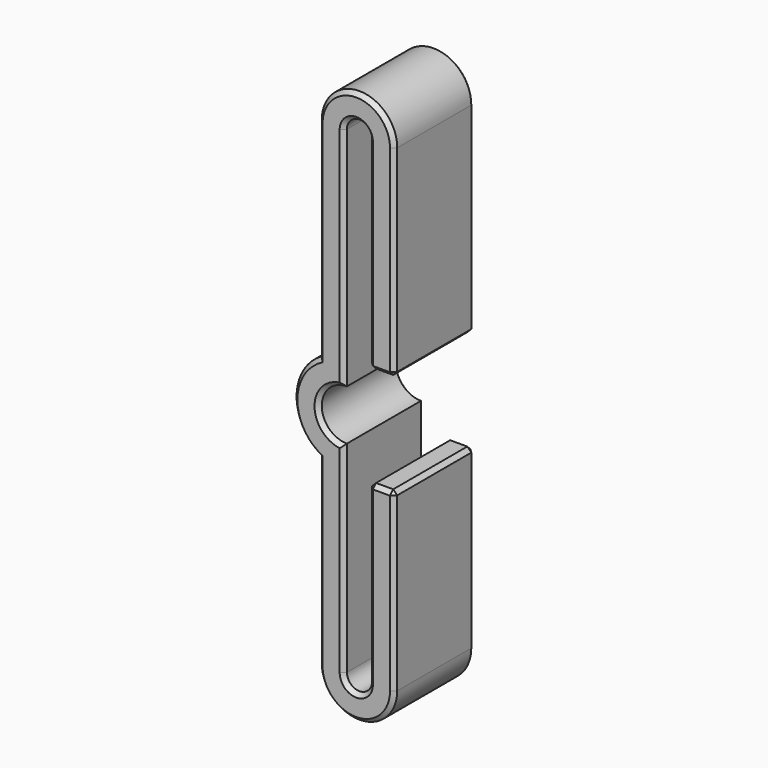
from build123d import *

# Parameters (mm, degrees)
F1_DEPTH = 6.35
F2_SIZE  = 0.254


# Not quite as in the source:
# - a feature names something its author has since deleted; it is built from what else it names


with BuildPart() as f1:
    # F0 (on Front) → F1 (new body)
    with BuildSketch(Plane.XZ):
        with BuildLine():
            Line((0, 1.5875), (0, 15.875))
            ThreePointArc((0, 15.875), (0.79375, 16.66875), (1.5875, 15.875))
            Line((1.5875, 15.875), (1.5875, 3.175))
            Line((1.5875, 3.175), (3.175, 3.175))
            Line((3.175, 3.175), (3.175, 15.875))
            ThreePointArc((3.175, 15.875), (0.79375, 18.25625), (-1.5875, 15.875))
            Line((-1.5875, 15.875), (-1.5875, 2.749630657))
            ThreePointArc((-1.5875, 2.749630657), (-3.175, 0), (-1.5875, -2.749630657))
            Line((-1.5875, -2.749630657), (-1.5875, -14.2875))
            ThreePointArc((-1.5875, -14.2875), (0.79375, -16.66875), (3.175, -14.2875))
            Line((3.175, -14.2875), (3.175, -3.175))
            Line((3.175, -3.175), (1.5875, -3.175))
            Line((1.5875, -3.175), (1.5875, -14.2875))
            ThreePointArc((1.5875, -14.2875), (0.79375, -15.08125), (0, -14.2875))
            Line((0, -14.2875), (0, -1.5875))
            ThreePointArc((0, -1.5875), (-1.5875, 0), (0, 1.5875))
        make_face()
    extrude(amount=F1_DEPTH)

    # F2
    f2_edges = [f1.edges().sort_by_distance(p)[0] for p in [
        (-1.5875, -6.35, 9.312315),
        (0.79375, -6.35, 18.25625),
        (3.175, -6.35, 9.525),
        (-3.175, -6.35, 0),
        (-1.5875, -6.35, -8.518565),
        (0.79375, -6.35, -16.66875),
        (3.175, -6.35, -8.73125),
        (2.38125, -6.35, 3.175),
        (2.38125, -6.35, -3.175),
        (0, -6.35, -7.9375),
        (-1.5875, -6.35, 0),
        (0, -6.35, 8.73125),
        (1.5875, -3.175, 3.175),
        (1.5875, -3.175, -3.175),
        (2.38125, 0, -3.175),
        (3.175, -3.175, -3.175),
        (2.38125, 0, 3.175),
        (3.175, -3.175, 3.175),
        (3.175, 0, 9.525),
        (3.175, 0, -8.73125),
        (-3.175, 0, 0),
        (1.5875, 0, -8.73125),
        (1.5875, 0, 9.525),
        (-1.5875, 0, 0),
    ]]
    chamfer(f2_edges, length=F2_SIZE)


solid = f1.part
